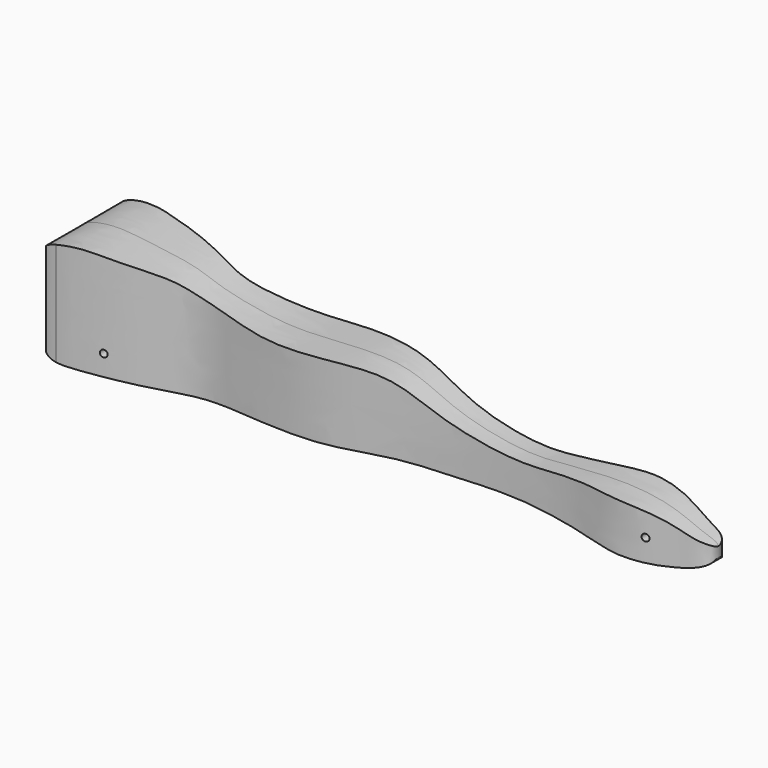
from build123d import *

# Parameters (mm, degrees)
F4_DEPTH = 22.225
F5_START = 17.562848
F5_DEPTH = 50.074789
F6_START = -92.075
F2_R     = 9.525
F6_DEPTH = 60.325
F3_R     = 1.5875
F7_DEPTH = 25.4


with BuildPart() as f4:
    # F0 (on Front) → F4 (new body, symmetric)
    with BuildSketch(Plane.XZ):
        with BuildLine():
            add(Edge.make_bspline(
                [(-146.05, -10.692352), (-145.642615, -6.266576), (-146.444901, -0.6892), (-145.418891, 9.304623), (-147.916358, 14.84784), (-132.008259, 18.469233), (-118.050036, 16.446484), (-94.767234, 14.138402), (-83.717757, 9.054911), (-64.192785, 4.974754), (-41.870685, 2.488918), (1.485559, 7.992714), (24.364791, -6.633507), (57.086507, -12.80712), (74.833543, -11.400202), (101.990603, -8.864215), (125.538144, -11.689836), (138.726142, -18.451973), (147.216841, -20.263843), (146.215218, -26.281661), (144.57663, -28.64875), (129.662446, -33.408048), (97.16568, -31.944528), (61.581863, -26.384998), (32.337613, -27.749954), (10.300403, -27.136991), (-10.43849, -28.578742), (-29.619868, -30.237379), (-63.427701, -30.280117), (-89.405822, -32.092524), (-112.755848, -31.672559), (-132.234581, -31.74417), (-150.087305, -31.815862), (-146.576335, -16.41039), (-146.05, -10.692352)],
                knots=[0, 0, 0, 0, 0.023682, 0.046035, 0.060753, 0.086902, 0.115995, 0.150295, 0.175913, 0.207065, 0.242308, 0.289056, 0.327175, 0.367806, 0.398806, 0.436349, 0.471889, 0.499782, 0.519075, 0.534577, 0.546095, 0.572773, 0.614748, 0.658876, 0.697892, 0.731843, 0.764225, 0.796253, 0.838213, 0.875766, 0.910476, 0.94332, 0.969403, 1, 1, 1, 1], degree=3))
        make_face()
    extrude(amount=F4_DEPTH, both=True)

    # F1 (on Top) → F5 (intersect)
    with BuildSketch(Plane.XY.offset(F5_START)):
        with BuildLine():
            add(Edge.make_bspline(
                [(-146.05, 0), (-146.05, 8.375908), (-145.598219, 21.739636), (-145.722062, 21.8687), (-139.127767, 23.05328), (-107.023731, 18.334878), (-83.679712, 9.351539), (-57.872861, 13.977602), (-22.353295, 15.873772), (9.122467, 8.962677), (53.865874, 7.142051), (89.052233, 7.953522), (107.96945, 13.090778), (126.121755, 9.122724), (135.249981, 6.571878), (146.05, 5.078349), (146.05, 0)],
                knots=[0, 0, 0, 0, 0.074887, 0.077288, 0.111524, 0.203654, 0.285335, 0.365778, 0.460487, 0.552364, 0.660191, 0.755329, 0.825823, 0.892361, 0.945096, 1, 1, 1, 1], degree=3))
            add(Edge.make_bspline(
                [(-146.05, 0), (-146.05, -8.375908), (-145.598219, -21.739636), (-145.722062, -21.8687), (-143.845847, -22.205738), (-141.136327, -22.225)],
                knots=[0, 0, 0, 0, 0.074887, 0.077288, 0.111524, 0.111524, 0.111524, 0.111524], degree=3))
            Line((-141.136327, -22.225), (-140.591541, -22.225))
            add(Edge.make_bspline(
                [(-140.591541, -22.225), (-133.154337, -22.174719), (-106.817772, -18.25562), (-83.679712, -9.351539), (-57.872861, -13.977602), (-22.353295, -15.873772), (9.122467, -8.962677), (53.865874, -7.142051), (89.052233, -7.953522), (107.96945, -13.090778), (126.121755, -9.122724), (135.249981, -6.571878), (146.05, -5.078349), (146.05, 0)],
                knots=[0.113767, 0.113767, 0.113767, 0.113767, 0.203654, 0.285335, 0.365778, 0.460487, 0.552364, 0.660191, 0.755329, 0.825823, 0.892361, 0.945096, 1, 1, 1, 1], degree=3))
        make_face()
        with BuildLine():
            Line((-140.591541, -22.225), (-141.136327, -22.225))
            add(Edge.make_bspline(
                [(-141.136327, -22.225), (-140.958789, -22.226262), (-140.777146, -22.226255), (-140.591541, -22.225)],
                knots=[0.111524, 0.111524, 0.111524, 0.111524, 0.113767, 0.113767, 0.113767, 0.113767], degree=3))
        make_face()
    extrude(amount=-F5_DEPTH, mode=Mode.INTERSECT)

    # F2 (on Right) → F6 (cut)
    with BuildSketch(Plane.YZ.offset(F6_START)):
        Circle(F2_R)
    extrude(amount=-F6_DEPTH, mode=Mode.SUBTRACT)

    # F3 (on Front) → F7 (cut, symmetric)
    with BuildSketch(Plane.XZ):
        with Locations((-120.65, -22.225)):
            Circle(F3_R)
        with Locations((120.65, -22.225)):
            Circle(F3_R)
    extrude(amount=F7_DEPTH, both=True, mode=Mode.SUBTRACT)


solid = f4.part
